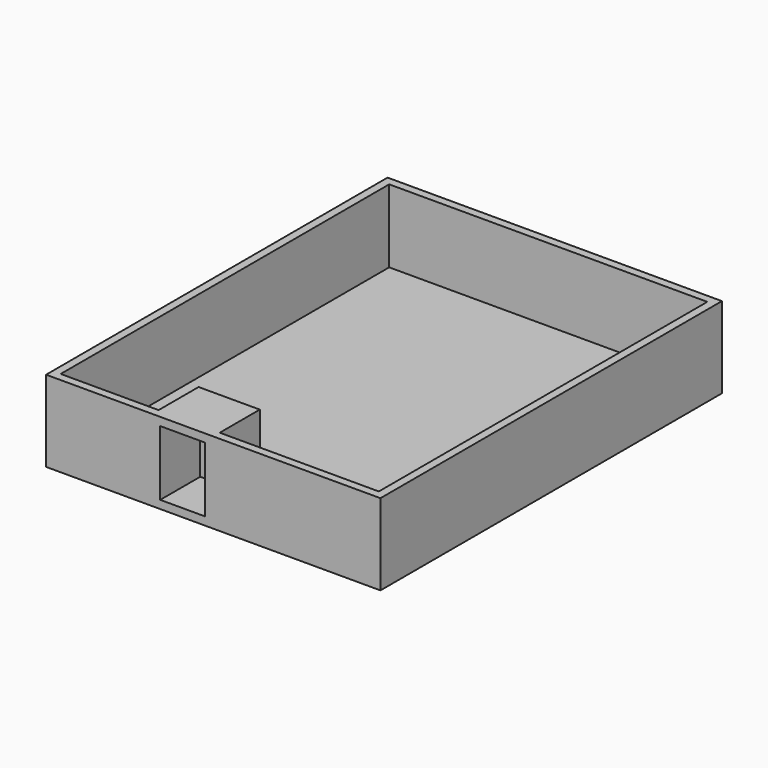
from build123d import *

# Parameters (mm, degrees)
F0_W         = 104.6088039875
F0_H         = 133.5426568985
F1_DEPTH     = 25.4
F2_T         = -2.54
F3_W         = 19.131584093
F3_H         = 25.4
F4_DEPTH     = 18.1840639561
F5_T         = 2.54
F5_T3_DEPTH  = 27.94
F5_T5_DEPTH  = 133.5426568985
F5_T7_DEPTH  = 104.6088039875
F5_T9_DEPTH  = 54.8444019938
F5_T11_DEPTH = 20.7240639561
F5_T13_DEPTH = 24.211584093
F5_T15_DEPTH = 35.7128179008


# Not quite as in the source:
# - a shell that OpenCascade refuses in one call is made with other operations: the cavity is built on its own and cut out


with BuildPart() as f1:
    # F0 (on Top) → F1 (new body)
    with BuildSketch(Plane.XY):
        with Locations((0, -9.2112720013)):
            Rectangle(F0_W, F0_H)
    extrude(amount=F1_DEPTH)

    # F2
    f2_openings = [f1.faces().sort_by_distance(p)[0] for p in [
        (0, -9.211272, 25.4),
    ]]
    offset(amount=F2_T, openings=f2_openings)

    # F3 (on face) → F4 (join)
    with BuildSketch(Plane.XZ.offset(75.9826004505)):
        with Locations((-9.5657920465, 12.7)):
            Rectangle(F3_W, F3_H)
    extrude(amount=-F4_DEPTH)

    # F5: shell of thickness 2.54, made by hand


with BuildPart() as f5_core1:
    # F5_t2: copy of F1
    add(f1.part)

    # the walls: a layer under each face that stays
    f5_faces = [f5_core1.faces().sort_by_distance(p)[0] for p in [
        (52.3044019938, -9.2112720013, 12.7),
        (-14.9441148554, -66.4438392435, 25.4),
        (49.7644019938, -9.2112720013, 13.97),
        (0, -9.2112720013, 2.54),
        (0, 55.020056448, 13.97),
        (-49.7644019938, -9.2112720013, 13.97),
        (-34.4479930434, -73.4426004505, 13.97),
        (-19.131584093, -65.6205684724, 13.97),
        (-9.5657920465, -57.7985364944, 13.97),
        (0, -65.6205684724, 13.97),
        (24.8822009969, -73.4426004505, 13.97),
        (-52.3044019938, -9.2112720013, 12.7),
        (0, -9.2112720013, 0),
        (0, 57.560056448, 12.7),
    ]]
    thicken(f5_faces, amount=-F5_T, mode=Mode.SUBTRACT)

    # F5_s4 → F5_t3 (cut)
    with BuildSketch(Plane.XY):
        Polygon((49.7390019938, 54.994656448), (52.3044019938, 55.020056448), (52.3044019938, 57.560056448), (49.7644019938, 57.560056448), align=None)
        Polygon((49.7390019938, -73.4172004505), (52.3044019938, -73.4426004505), (52.3044019938, -75.9826004505), (49.7644019938, -75.9826004505), align=None)
        Polygon((-49.7390019938, 54.994656448), (-49.7644019938, 57.560056448), (-52.3044019938, 57.560056448), (-52.3044019938, 55.020056448), align=None)
        Polygon((-49.7390019938, -73.4172004505), (-52.3044019938, -73.4426004505), (-52.3044019938, -75.9826004505), (-49.7644019938, -75.9826004505), align=None)
        Polygon((-19.156984093, -73.4172004505), (-19.131584093, -75.9826004505), (-16.591584093, -75.9826004505), (-16.591584093, -73.4426004505), align=None)
        Polygon((0.0254, -73.4172004505), (-2.54, -73.4426004505), (-2.54, -75.9826004505), (0, -75.9826004505), align=None)
    extrude(amount=F5_T3_DEPTH, mode=Mode.SUBTRACT)

    # F5_s6 → F5_t5 (cut)
    with BuildSketch(Plane.XZ.offset(-57.560056448)):
        Polygon((49.7390019938, 2.5654), (52.3044019938, 2.54), (52.3044019938, 0), (49.7644019938, 0), align=None)
        Polygon((-49.7390019938, 2.5654), (-49.7644019938, 0), (-52.3044019938, 0), (-52.3044019938, 2.54), align=None)
    extrude(amount=F5_T5_DEPTH, mode=Mode.SUBTRACT)

    # F5_s8 → F5_t7 (cut)
    with BuildSketch(Plane.YZ.offset(-52.3044019938)):
        Polygon((54.994656448, 2.5654), (55.020056448, 0), (57.560056448, 0), (57.560056448, 2.54), align=None)
    extrude(amount=F5_T7_DEPTH, mode=Mode.SUBTRACT)

    # F5_s10 → F5_t9 (cut)
    with BuildSketch(Plane.YZ.offset(-2.54)):
        Polygon((-73.4172004505, 2.5654), (-73.4426004505, 0), (-75.9826004505, 0), (-75.9826004505, 2.54), align=None)
    extrude(amount=F5_T9_DEPTH, mode=Mode.SUBTRACT)

    # F5_s12 → F5_t11 (cut)
    with BuildSketch(Plane.XZ.offset(55.2585364944)):
        Polygon((0.0254, 2.5654), (0, 0), (-2.54, 0), (-2.54, 2.54), align=None)
        Polygon((-19.156984093, 2.5654), (-19.131584093, 0), (-16.591584093, 0), (-16.591584093, 2.54), align=None)
    extrude(amount=F5_T11_DEPTH, mode=Mode.SUBTRACT)

    # F5_s14 → F5_t13 (cut)
    with BuildSketch(Plane.YZ.offset(-21.671584093)):
        Polygon((-57.7731364944, 2.5654), (-57.7985364944, 0), (-60.3385364944, 0), (-60.3385364944, 2.54), align=None)
    extrude(amount=F5_T13_DEPTH, mode=Mode.SUBTRACT)

    # F5_s16 → F5_t15 (cut)
    with BuildSketch(Plane.YZ.offset(-52.3044019938)):
        Polygon((-73.4172004505, 2.5654), (-73.4426004505, 0), (-75.9826004505, 0), (-75.9826004505, 2.54), align=None)
    extrude(amount=F5_T15_DEPTH, mode=Mode.SUBTRACT)


with BuildPart() as f1_1:
    add(f1.part)

    # what is left inside the walls is the cavity
    f5_cavity = [f5_core1.part.solids().sort_by_distance(p)[0] for p in [
        (-2.5654, -65.553224, 12.7),
    ]]
    add(f5_cavity, mode=Mode.SUBTRACT)


solid = f1_1.part
